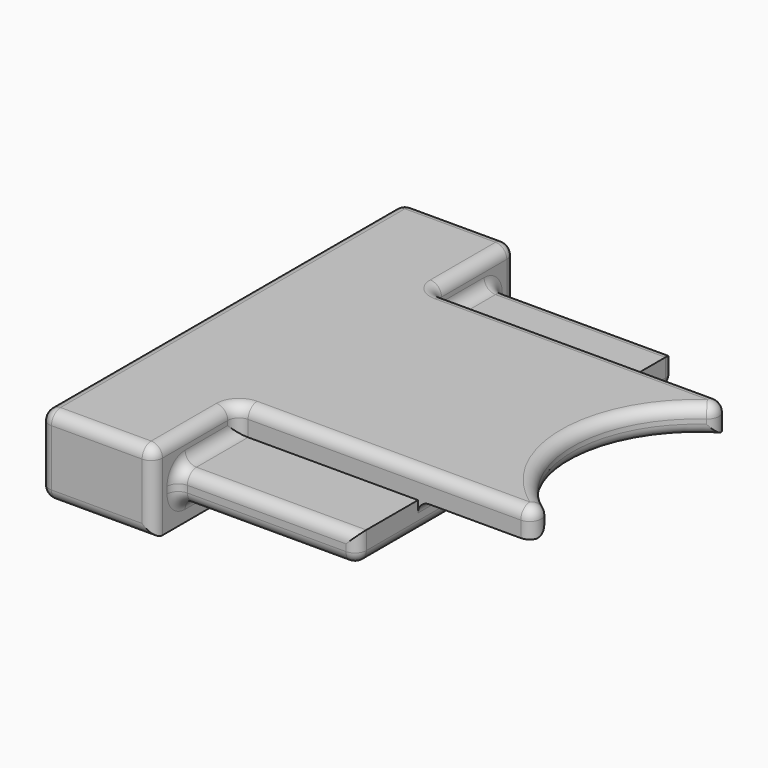
from build123d import *

# Parameters (mm, degrees)
F1_DEPTH = 16
F2_W     = 20
F2_H     = 3.5
F3_DEPTH = 5
F5_DEPTH = 5
F6_W     = 17.5
F6_H     = 1.3
F7_DEPTH = 8
F8_R     = 0.5


# Not quite as in the source:
# - ends of sketch curves that miss each other by under 0.0002 mm in the source are joined


with BuildPart() as f1:
    # F0 (on Right) → F1 (new body)
    with BuildSketch(Plane.YZ):
        Polygon((14.15, 1.3), (14.15, 2.5), (3.35, 2.5), (3.35, 1.3), (0, 1.3), (0, 0), (17.5, 0), (17.5, 1.3), align=None)
    extrude(amount=F1_DEPTH)

    # F2 (on face) → F3 (join)
    with BuildSketch(Plane(origin=(0, 0, 0), x_dir=(0, -1, 0), z_dir=(-1, 0, 0))):
        with Locations((-8.75, 0.75)):
            Rectangle(F2_W, F2_H)
    extrude(amount=F3_DEPTH)

    # F4 (on face) → F5 (cut)
    with BuildSketch(Plane.XY.offset(2.5)):
        with BuildLine():
            ThreePointArc((16.0075383861, 14.2499948339), (10.5000136527, 8.7377452223), (16.0320477827, 3.2500933699))
            Line((16.0320477827, 3.2500933699), (16.0075383861, 14.2499948339))
        make_face()
    extrude(amount=-F5_DEPTH, mode=Mode.SUBTRACT)

    # F6 (on face) → F7 (cut)
    with BuildSketch(Plane.YZ.offset(16)):
        with Locations((8.75, 0.65)):
            Rectangle(F6_W, F6_H)
    extrude(amount=-F7_DEPTH, mode=Mode.SUBTRACT)

    # F8
    f8_edges = [f1.edges().sort_by_distance(p)[0] for p in [
        (7.477985, 3.35, 2.5),
        (14.955969, 3.35, 1.9),
        (14.955969, 14.15, 1.9),
        (10.5, 8.75, 2.5),
        (10.5, 8.75, 1.3),
        (7.477985, 14.15, 2.5),
        (8, 8.75, 1.3),
        (0, 8.75, 0),
        (0, 1.675, 1.3),
        (0, 0, 0.65),
        (0, 17.5, 0.65),
        (0, 15.825, 1.3),
        (-5, 8.75, -1),
        (-5, -1.25, 0.75),
        (-5, 8.75, 2.5),
        (-5, 18.75, 0.75),
        (-2.5, -1.25, -1),
        (-2.5, -1.25, 2.5),
        (0, -1.25, 0.75),
        (-2.5, 18.75, 2.5),
        (-2.5, 18.75, -1),
        (0, 18.75, 0.75),
        (4, 17.5, 1.3),
        (8, 17.5, 0.65),
        (4, 17.5, 0),
        (4, 0, 0),
        (8, 0, 0.65),
        (4, 0, 1.3),
        (8, 8.75, 0),
        (0, 1.05, 2.5),
        (0, 16.45, 2.5),
        (0, 3.35, 1.9),
        (0, 14.15, 1.9),
    ]]
    fillet(f8_edges, radius=F8_R)


solid = f1.part
